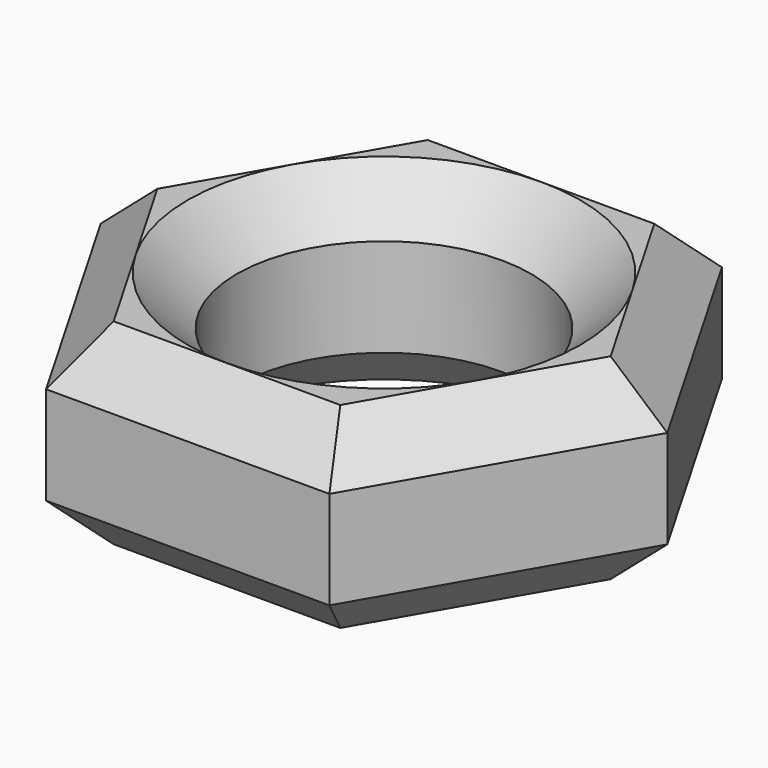
from build123d import *

# Parameters (mm, degrees)
F1_DEPTH = 20
F2_R     = 15
F3_DEPTH = 25
F4_SIZE  = 4.99999


# Not quite as in the source:
# - a fillet or chamfer is up to 0.001 mm smaller than in the source, because OpenCascade refuses the exact size


with BuildPart() as f1:
    # F0 (on Top) → F1 (new body)
    with BuildSketch(Plane.XY):
        Polygon((14.4337567297, 25), (-14.4337567297, 25), (-28.8675134595, 0), (-14.4337567297, -25), (14.4337567297, -25), (28.8675134595, 0), align=None)
    extrude(amount=F1_DEPTH)

    # F2 (on face) → F3 (cut)
    with BuildSketch(Plane.XY.offset(20)):
        Circle(F2_R)
    extrude(amount=-F3_DEPTH, mode=Mode.SUBTRACT)

    # F4 (size 5 in the source; OpenCascade refuses exactly that, so slightly less here)
    f4_edges = [f1.edges().sort_by_distance(p)[0] for p in [
        (0, 25, 20),
        (21.650635, 12.5, 20),
        (-21.650635, 12.5, 20),
        (21.650635, -12.5, 20),
        (-21.650635, -12.5, 20),
        (0, -25, 20),
        (-15, 0, 20),
        (0, 25, 0),
        (21.650635, 12.5, 0),
        (-21.650635, 12.5, 0),
        (21.650635, -12.5, 0),
        (-21.650635, -12.5, 0),
        (0, -25, 0),
        (-15, 0, 0),
    ]]
    chamfer(f4_edges, length=F4_SIZE)


solid = f1.part
